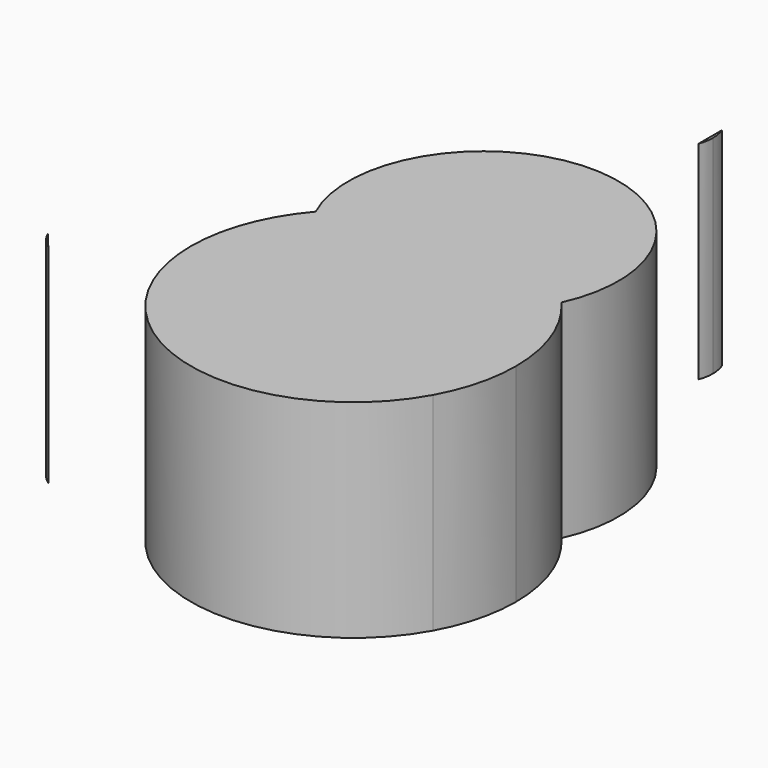
from build123d import *

# Parameters (mm, degrees)
F1_DEPTH = 30


with BuildPart() as f1:
    # F0 (on Top) → F1 (new body)
    with BuildSketch(Plane.XY):
        with BuildLine():
            ThreePointArc((-7.1621949879, 10.849099638), (-6.1600107613, -11.4478935801), (13, 0))
            ThreePointArc((13, 0), (11.4478935801, 6.1600107613), (7.1621949879, 10.849099638))
            ThreePointArc((7.1621949879, 10.849099638), (0, 8.9623826913), (-7.1621949879, 10.849099638))
        make_face()
        with BuildLine():
            ThreePointArc((7.1621949879, 10.849099638), (11.4478935801, 6.1600107613), (13, 0))
            ThreePointArc((13, 0), (-6.1600107613, -11.4478935801), (-7.1621949879, 10.849099638))
            ThreePointArc((-7.1621949879, 10.849099638), (-10.0406665828, 12.9868020286), (-12.3083921231, 15.763993255))
            ThreePointArc((-12.3083921231, 15.763993255), (-8.7701812278, -17.9745353551), (20, 0))
            ThreePointArc((20, 0), (17.9745353551, 8.7701812278), (12.3083921231, 15.763993255))
            ThreePointArc((12.3083921231, 15.763993255), (10.0406665828, 12.9868020286), (7.1621949879, 10.849099638))
        make_face()
        with BuildLine():
            ThreePointArc((-7.1621949879, 10.849099638), (0, 8.9623826913), (7.1621949879, 10.849099638))
            ThreePointArc((7.1621949879, 10.849099638), (0, 13), (-7.1621949879, 10.849099638))
        make_face()
        with BuildLine():
            ThreePointArc((-7.1621949879, 10.849099638), (0, 13), (7.1621949879, 10.849099638))
            ThreePointArc((7.1621949879, 10.849099638), (10.0406665828, 12.9868020286), (12.3083921231, 15.763993255))
            ThreePointArc((12.3083921231, 15.763993255), (0, 20), (-12.3083921231, 15.763993255))
            ThreePointArc((-12.3083921231, 15.763993255), (-10.0406665828, 12.9868020286), (-7.1621949879, 10.849099638))
        make_face()
        with BuildLine():
            ThreePointArc((13.8247061586, 19.0033549572), (13.1665512762, 17.336864069), (12.3083921231, 15.763993255))
            ThreePointArc((12.3083921231, 15.763993255), (17.9745353551, 8.7701812278), (20, 0))
            ThreePointArc((20, 0), (-8.7701812278, -17.9745353551), (-12.3083921231, 15.763993255))
            ThreePointArc((-12.3083921231, 15.763993255), (-13.1665512762, 17.336864069), (-13.8247061586, 19.0033549572))
            ThreePointArc((-13.8247061586, 19.0033549572), (-15.9007698993, 17.3036272674), (-17.7695516679, 15.3783299979))
            ThreePointArc((-17.7695516679, 15.3783299979), (-22.0208363169, 8.2056546297), (-23.5, 0))
            ThreePointArc((-23.5, 0), (-22.7597361756, -5.851872283), (-20.5855821944, -11.3350697272))
            ThreePointArc((-20.5855821944, -11.3350697272), (0, -23.5), (20.5855821944, -11.3350697272))
            ThreePointArc((20.5855821944, -11.3350697272), (22.7597361756, -5.851872283), (23.5, 0))
            ThreePointArc((23.5, 0), (22.0208363169, 8.2056546297), (17.7695516679, 15.3783299979))
            ThreePointArc((17.7695516679, 15.3783299979), (15.9007698993, 17.3036272674), (13.8247061586, 19.0033549572))
        make_face()
        with BuildLine():
            ThreePointArc((-12.3083921231, 15.763993255), (0, 20), (12.3083921231, 15.763993255))
            ThreePointArc((12.3083921231, 15.763993255), (13.1665512762, 17.336864069), (13.8247061586, 19.0033549572))
            ThreePointArc((13.8247061586, 19.0033549572), (3.6269971249, 23.2184170833), (-7.3703918295, 22.3142852066))
            ThreePointArc((-7.3703918295, 22.3142852066), (-10.7260714831, 20.9093613135), (-13.8247061586, 19.0033549572))
            ThreePointArc((-13.8247061586, 19.0033549572), (-13.1665512762, 17.336864069), (-12.3083921231, 15.763993255))
        make_face()
        with BuildLine():
            ThreePointArc((14.5376173087, 23.5), (14.3582834028, 21.2235960953), (13.8247061586, 19.0033549572))
            ThreePointArc((13.8247061586, 19.0033549572), (15.9007698993, 17.3036272674), (17.7695516679, 15.3783299979))
            ThreePointArc((17.7695516679, 15.3783299979), (17.7957261948, 31.5641564532), (5.6083085947, 42.2153777629))
            ThreePointArc((5.6083085947, 42.2153777629), (-0.2051065098, 43.0365406718), (-6, 42.093506665))
            ThreePointArc((-6, 42.093506665), (-17.8794033097, 31.3768919879), (-17.7695516679, 15.3783299979))
            ThreePointArc((-17.7695516679, 15.3783299979), (-15.9007698993, 17.3036272674), (-13.8247061586, 19.0033549572))
            ThreePointArc((-13.8247061586, 19.0033549572), (-2.2764039047, 37.8582834028), (14.5376173087, 23.5))
        make_face()
        with BuildLine():
            ThreePointArc((-7.3703918295, 22.3142852066), (3.6269971249, 23.2184170833), (13.8247061586, 19.0033549572))
            ThreePointArc((13.8247061586, 19.0033549572), (14.3582834028, 21.2235960953), (14.5376173087, 23.5))
            ThreePointArc((14.5376173087, 23.5), (-2.2764039047, 37.8582834028), (-13.8247061586, 19.0033549572))
            ThreePointArc((-13.8247061586, 19.0033549572), (-10.7260714831, 20.9093613135), (-7.3703918295, 22.3142852066))
        make_face()
    extrude(amount=F1_DEPTH)


with BuildPart() as f1b:
    # F0 (on Top) → F1, piece 2 (new body)
    with BuildSketch(Plane.XY):
        with BuildLine():
            Line((5.6083085947, 59.5858506858), (5.6083085947, 55.321170296))
            ThreePointArc((5.6083085947, 55.321170296), (5.9012647614, 56.3695020887), (6, 57.4535104909))
            ThreePointArc((6, 57.4535104909), (5.9012647614, 58.5375188931), (5.6083085947, 59.5858506858))
        make_face()
    extrude(amount=F1_DEPTH)


with BuildPart() as f1c:
    # F0 (on Top) → F1, piece 3 (new body)
    with BuildSketch(Plane.XY):
        with BuildLine():
            ThreePointArc((-38.0529754103, -7.6076154565), (-37.1602081866, -9.1142838858), (-35.8704063618, -10.2989755437))
            ThreePointArc((-35.8704063618, -10.2989755437), (-36.9865719452, -8.9734728929), (-38.0529754103, -7.6076154565))
        make_face()
    extrude(amount=F1_DEPTH)


solid = Compound([f1.part, f1b.part, f1c.part])
